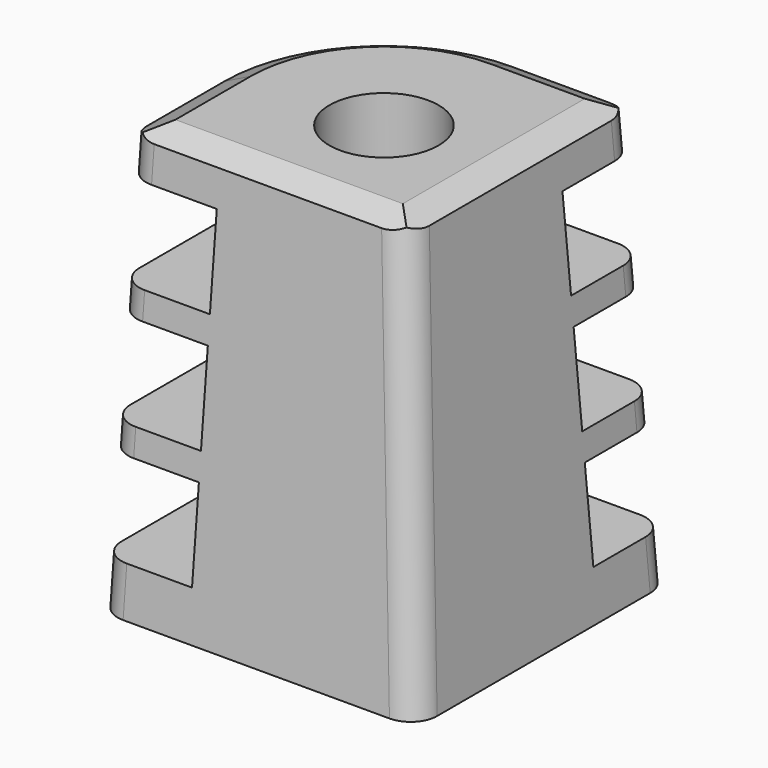
from build123d import *

# Parameters (mm, degrees)
F0_W          = 24
F0_H          = 24
F1_DEPTH      = 3.6
F2_R          = 4.3
F2_R_2        = 2.25
F3_DEPTH      = 4.5
F4_DEPTH      = 10
F5_R          = 2.25
F6_DEPTH      = 6.7
F7_W          = 17.1
F7_H          = 17.1
F7_R          = 2.25
F8_DEPTH      = 2
F9_W          = 17.1
F9_H          = 17.1
F9_R          = 2.25
F10_DEPTH     = 6.7
F11_W         = 17.1
F11_H         = 17.1
F11_R         = 2.25
F12_DEPTH     = 2
F13_W         = 17.1
F13_H         = 17.1
F14_DEPTH     = 6.7
F15_W         = 24
F15_H         = 24
F16_DEPTH     = 3.4
F17_R         = 5.1
F18_R         = 12
F19_R         = 4.1
F20_DEPTH     = 23
F23_DEPTH     = 25
F24_DEPTH     = 25
F25_DEPTH     = 50
F26_T1_DEPTH  = 14.1796577476
F26_T3_DEPTH  = 30.9358787863
F26_T5_DEPTH  = 30.9358787863
F26_T7_DEPTH  = 14.1796577476
F26_T10_ANGLE = 90
F27_R         = 2
F28_R         = 2
F29_R         = 2


# Not quite as in the source:
# - a fillet or chamfer that OpenCascade refuses, or shapes differently, is made with other operations: its cross-section is extruded or revolved along the edge and cut away or added


with BuildPart() as f1:
    # F0 (on Top) → F1 (new body)
    with BuildSketch(Plane.XY):
        with Locations((12, 12)):
            Rectangle(F0_W, F0_H)
    extrude(amount=F1_DEPTH)

    # F2 (on face) → F3 (join)
    with BuildSketch(Plane(origin=(0, 0, 0), x_dir=(1, 0, 0), z_dir=(0, 0, -1))):
        with Locations((12, -12)):
            Circle(F2_R)
        with Locations((12, -12)):
            Circle(F2_R_2, mode=Mode.SUBTRACT)
    extrude(amount=F3_DEPTH)

    # F4 (cut): a face of the model
    f4_faces = [f1.faces().sort_by_distance(p)[0] for p in [
        (12, 12, 0),
    ]]
    extrude(f4_faces, amount=-F4_DEPTH, mode=Mode.SUBTRACT)

    # F5 (on face) → F6 (join)
    with BuildSketch(Plane.XY.offset(3.6)):
        Polygon((6.9, 0), (20, 0), (24, 0), (24, 17.1), (6.9, 17.1), align=None)
        with Locations((12, 12)):
            Circle(F5_R, mode=Mode.SUBTRACT)
    extrude(amount=F6_DEPTH)

    # F7 (on face) → F8 (join)
    with BuildSketch(Plane.XY.offset(10.3)):
        Polygon((0, 24), (0, 0), (6.9, 0), (6.9, 17.1), (24, 17.1), (24, 24), align=None)
        with Locations((15.45, 8.55)):
            Rectangle(F7_W, F7_H)
        with Locations((12, 12)):
            Circle(F7_R, mode=Mode.SUBTRACT)
    extrude(amount=F8_DEPTH)

    # F9 (on face) → F10 (join)
    with BuildSketch(Plane.XY.offset(12.3)):
        with Locations((15.45, 8.55)):
            Rectangle(F9_W, F9_H)
        with Locations((12, 12)):
            Circle(F9_R, mode=Mode.SUBTRACT)
    extrude(amount=F10_DEPTH)

    # F11 (on face) → F12 (join)
    with BuildSketch(Plane.XY.offset(19)):
        Polygon((0, 0), (6.9, 0), (6.9, 17.1), (24, 17.1), (24, 24), (0, 24), align=None)
        with Locations((15.45, 8.55)):
            Rectangle(F11_W, F11_H)
        with Locations((12, 12)):
            Circle(F11_R, mode=Mode.SUBTRACT)
    extrude(amount=F12_DEPTH)

    # F13 (on face) → F14 (join)
    with BuildSketch(Plane.XY.offset(21)):
        with Locations((15.45, 8.55)):
            Rectangle(F13_W, F13_H)
    extrude(amount=F14_DEPTH)

    # F15 (on face) → F16 (join)
    with BuildSketch(Plane.XY.offset(27.7)):
        with Locations((12, 12)):
            Rectangle(F15_W, F15_H)
    extrude(amount=F16_DEPTH)

    # F17
    f17_edges = [f1.edges().sort_by_distance(p)[0] for p in [
        (6.9, 17.1, 6.95),
        (6.9, 17.1, 15.65),
        (6.9, 17.1, 24.35),
    ]]
    fillet(f17_edges, radius=F17_R)

    # F18
    f18_edges = [f1.edges().sort_by_distance(p)[0] for p in [
        (0, 24, 11.3),
        (0, 24, 20),
        (0, 24, 29.4),
    ]]
    fillet(f18_edges, radius=F18_R)

    # F19 (on face) → F20 (cut)
    with BuildSketch(Plane.XY.offset(31.1)):
        with Locations((12, 12)):
            Circle(F19_R)
    extrude(amount=-F20_DEPTH, mode=Mode.SUBTRACT)

    # F21 (on face) → F23 (join)
    with BuildSketch(Plane.YZ.offset(24)):
        Polygon((0, 31.1), (0, 0), (3, 31.1), align=None)
    extrude(amount=F23_DEPTH)

    # F22 (on face) → F24 (cut)
    with BuildSketch(Plane.XZ):
        Polygon((21, 31.1), (24, 0), (24, 31.1), align=None)
    extrude(amount=-F24_DEPTH, mode=Mode.SUBTRACT)

    # F25 (cut): a face of the model
    f25_faces = [f1.faces().sort_by_distance(p)[0] for p in [
        (49, 1, 20.7333333333),
    ]]
    extrude(f25_faces, amount=-F25_DEPTH, mode=Mode.SUBTRACT)

    # F26: chamfer of 1 x 2 on 5 edges, made by hand

    # F26_s2 → F26_t1 (cut)
    with BuildSketch(Plane.XZ.offset(-12)):
        Polygon((2, 31.1), (0, 30.1), (0, 31.1), align=None)
    extrude(amount=F26_T1_DEPTH, mode=Mode.SUBTRACT)

    # F26_s4 → F26_t3 (cut)
    with BuildSketch(Plane.YZ.offset(-4.9679393932)):
        Polygon((2.9220612214, 30.2920346615), (4.912820546, 31.1), (3, 31.1), align=None)
    extrude(amount=F26_T3_DEPTH, mode=Mode.SUBTRACT)

    # F26_s6 → F26_t5 (cut)
    with BuildSketch(Plane.XZ.offset(-28.9679393932)):
        Polygon((21.0779387786, 30.2920346615), (19.087179454, 31.1), (21, 31.1), align=None)
    extrude(amount=F26_T5_DEPTH, mode=Mode.SUBTRACT)

    # F26_s8 → F26_t7 (cut)
    with BuildSketch(Plane.YZ.offset(12)):
        Polygon((24, 30.1), (22, 31.1), (24, 31.1), align=None)
    extrude(amount=F26_T7_DEPTH, mode=Mode.SUBTRACT)

    # F26_s9 → F26_t10 (revolve, cut)
    with BuildSketch(Plane.YZ.offset(12)):
        Polygon((22, 31.1), (24, 30.1), (24, 31.1), align=None)
    revolve(axis=Axis((12, 12, 31.1), (0, 0, 1)), revolution_arc=F26_T10_ANGLE, mode=Mode.SUBTRACT)

    # F27
    f27_edges = [f1.edges().sort_by_distance(p)[0] for p in [
        (22.538969, 1.461031, 15.146017),
    ]]
    fillet(f27_edges, radius=F27_R)

    # F28
    f28_edges = [f1.edges().sort_by_distance(p)[0] for p in [
        (0, 2.787781, 28.9),
        (0, 1.92926, 20),
        (0, 1.090032, 11.3),
        (0, 0.173633, 1.8),
        (0, 24, 1.8),
        (23.826367, 24, 1.8),
        (22.909968, 24, 11.3),
        (22.07074, 24, 20),
        (21.212219, 24, 28.9),
    ]]
    fillet(f28_edges, radius=F28_R)

    # F29
    f29_edges = [f1.edges().sort_by_distance(p)[0] for p in [
        (7.7, 12, -4.5),
    ]]
    fillet(f29_edges, radius=F29_R)


solid = f1.part
